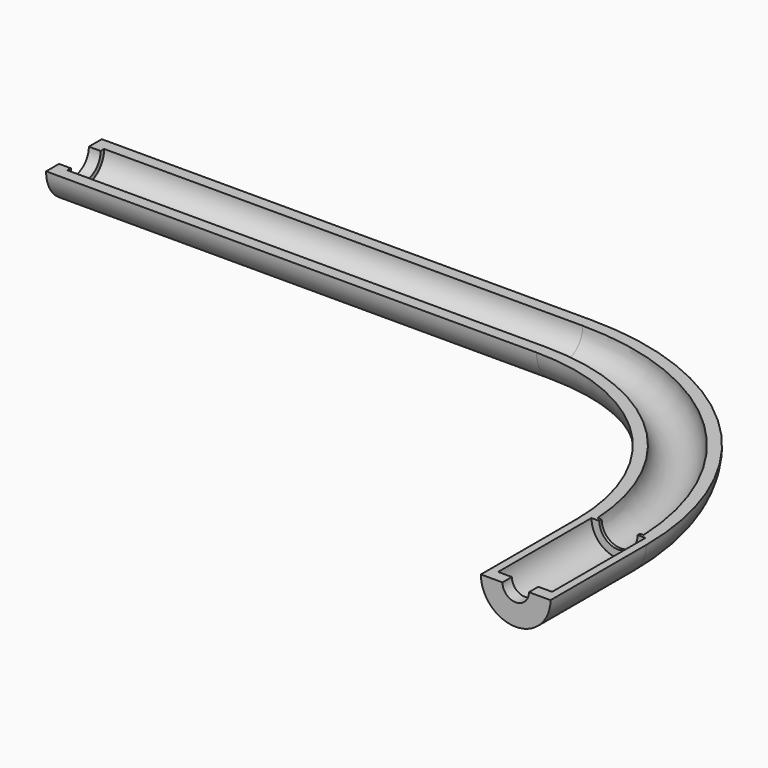
from build123d import *

# Parameters (mm, degrees)
F4_T      = -1.524
F6_DEPTH  = 1.524
F7_DEPTH  = 1.143
F9_DEPTH  = 1.524
F10_DEPTH = 13.97
F12_DEPTH = 1.524


with BuildPart() as f3:
    # F3: sweep along a path in F0
    with BuildLine(Plane.XY) as f3_path:
        ThreePointArc((93.98, -30.48), (85.0526146906, -8.9273853094), (63.5, 0))
        Line((63.5, 0), (0, 0))
    # F2 (on plane+point) → F3 (sweep)
    with BuildSketch(Plane.XZ.offset(30.48)):
        with BuildLine():
            Line((98.4885, 0), (89.4715, 0))
            ThreePointArc((89.4715, 0), (93.98, -4.5085), (98.4885, 0))
        make_face()
    sweep(path=f3_path.line)

    # F4
    f4_openings = [f3.faces().sort_by_distance(p)[0] for p in [
        (87.501546, -6.478454, 0),
    ]]
    offset(amount=F4_T, openings=f4_openings)

    # F5 (on face) → F6 (cut, through all)
    with BuildSketch(Plane.XZ.offset(30.48)):
        with BuildLine():
            ThreePointArc((91.5035, 0), (93.98, -2.4765), (96.4565, 0))
            Line((96.4565, 0), (91.5035, 0))
        make_face()
    extrude(amount=-F6_DEPTH, mode=Mode.SUBTRACT)

    # F5 (on face) → F7 (cut)
    with BuildSketch(Plane.XZ.offset(30.48)):
        with BuildLine():
            Line((97.4725, 0), (96.4565, 0))
            ThreePointArc((96.4565, 0), (93.98, -2.4765), (91.5035, 0))
            Line((91.5035, 0), (90.4875, 0))
            ThreePointArc((90.4875, 0), (93.98, -3.4925), (97.4725, 0))
        make_face()
    extrude(amount=-F7_DEPTH, mode=Mode.SUBTRACT)

    # F8 (on face) → F9 (cut, through all)
    with BuildSketch(Plane(origin=(0, 0, 0), x_dir=(0, -1, 0), z_dir=(-1, 0, 0))):
        with BuildLine():
            ThreePointArc((-2.413, 0), (0, -2.413), (2.413, 0))
            Line((2.413, 0), (-2.413, 0))
        make_face()
    extrude(amount=-F9_DEPTH, mode=Mode.SUBTRACT)

    # F5 (on face) → F10 (join)
    with BuildSketch(Plane.XZ.offset(30.48)):
        with BuildLine():
            Line((98.4885, 0), (97.4725, 0))
            ThreePointArc((97.4725, 0), (93.98, -3.4925), (90.4875, 0))
            Line((90.4875, 0), (89.4715, 0))
            ThreePointArc((89.4715, 0), (93.98, -4.5085), (98.4885, 0))
        make_face()
    extrude(amount=F10_DEPTH)

    # F11 (on face) → F12 (join)
    with BuildSketch(Plane.XZ.offset(44.45)):
        with BuildLine():
            Line((98.4885, 0), (97.4725, 0))
            ThreePointArc((97.4725, 0), (93.98, -3.4925), (90.4875, 0))
            Line((90.4875, 0), (89.4715, 0))
            ThreePointArc((89.4715, 0), (93.98, -4.5085), (98.4885, 0))
        make_face()
        with BuildLine():
            ThreePointArc((90.4875, 0), (93.98, -3.4925), (97.4725, 0))
            Line((97.4725, 0), (95.6945, 0))
            ThreePointArc((95.6945, 0), (93.98, -1.7145), (92.2655, 0))
            Line((92.2655, 0), (90.4875, 0))
        make_face()
    extrude(amount=F12_DEPTH)


solid = f3.part
